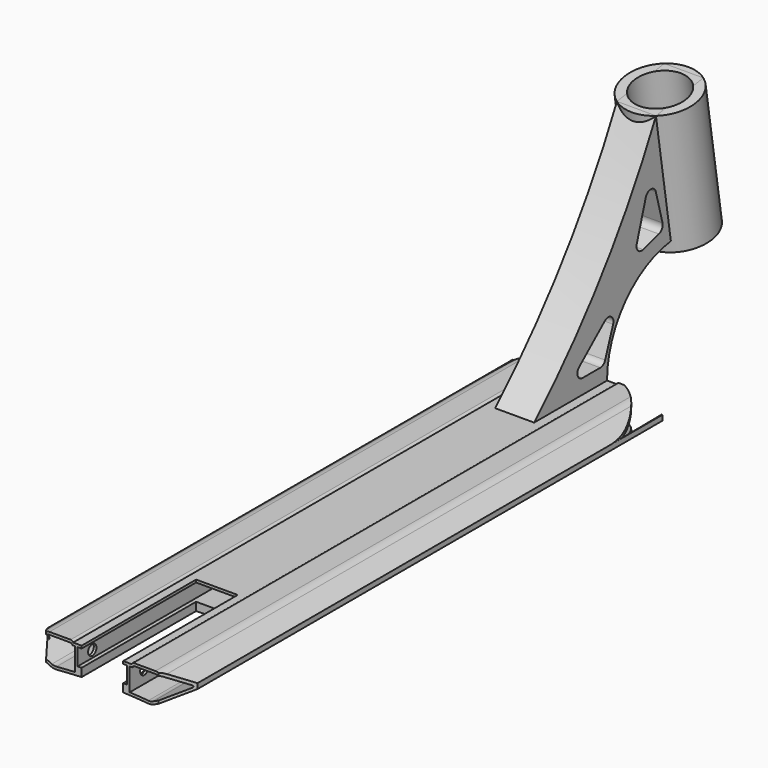
from build123d import *

# Parameters (mm, degrees)
F1_DEPTH       = 250
F2_W           = 38
F2_H           = 13
F3_DEPTH       = 250
F4_T1_DEPTH    = 509.3674969976
F5_R           = 9
F7_DEPTH       = 500.001
F9_DEPTH       = 0.9604886552
F9_DEPTH_BACK  = 22.8653446865
F11_DEPTH      = 0.9604887634
F11_DEPTH_BACK = 22.8653447865
F13_DEPTH      = 15
F14_R          = 27.5
F15_DEPTH      = 100
F17_D          = 40
F19_D          = 8
F19_DEPTH      = 78.501
F21_DEPTH      = 72.501


# Not quite as in the source:
# - a fillet or chamfer that OpenCascade refuses, or shapes differently, is made with other operations: its cross-section is extruded or revolved along the edge and cut away or added


with BuildPart() as f1:
    # F0 (on Front) → F1 (new body, symmetric)
    with BuildSketch(Plane.XZ):
        with BuildLine():
            Line((22.5, 21.5643446865), (0, 21.5643446865))
            Line((0, 21.5643446865), (-22.5, 21.5643446865))
            Line((-22.5, 21.5643446865), (-22.5, 22.8643446865))
            Line((-22.5, 22.8643446865), (-43.8217498065, 22.8643446865))
            Line((-43.8217498065, 22.8643446865), (-57.5, 12.151993139))
            Line((-57.5, 12.151993139), (-57.5, 8.151993139))
            Line((-57.5, 8.151993139), (-37.5, -1.1356553135))
            ThreePointArc((-37.5, -1.1356553135), (0, 0.564188832), (37.5, -1.1356553135))
            Line((37.5, -1.1356553135), (57.5, 8.151993139))
            Line((57.5, 8.151993139), (57.5, 12.151993139))
            Line((57.5, 12.151993139), (43.8217498065, 22.8643446865))
            Line((43.8217498065, 22.8643446865), (22.5, 22.8643446865))
            Line((22.5, 22.8643446865), (22.5, 21.5643446865))
        make_face()
    extrude(amount=F1_DEPTH, both=True)

    # F2 (on Front) → F3 (cut, symmetric)
    with BuildSketch(Plane.XZ):
        with Locations((0, 13.0643446865)):
            Rectangle(F2_W, F2_H)
    extrude(amount=F3_DEPTH, both=True, mode=Mode.SUBTRACT)

    # F4: fillet of radius 2 on 2 edges, made by hand

    # F4_s2 → F4_t1 (cut)
    with BuildSketch(Plane.XZ.offset(-254.6837484988)):
        with BuildLine():
            ThreePointArc((-24.3734993995, 22.8643446865), (-23.2333239744, 22.507512359), (-22.5, 21.5643446865))
            Line((-22.5, 21.5643446865), (-22.5, 22.8643446865))
            Line((-22.5, 22.8643446865), (-24.3734993995, 22.8643446865))
        make_face()
        with BuildLine():
            ThreePointArc((24.3734993995, 22.8643446865), (23.2333239744, 22.507512359), (22.5, 21.5643446865))
            Line((22.5, 21.5643446865), (22.5, 22.8643446865))
            Line((22.5, 22.8643446865), (24.3734993995, 22.8643446865))
        make_face()
    extrude(amount=F4_T1_DEPTH, mode=Mode.SUBTRACT)

    # F5
    f5_edges = [f1.edges().sort_by_distance(p)[0] for p in [
        (43.82175, 0, 22.864345),
        (-43.82175, 0, 22.864345),
        (-37.5, 0, -1.135655),
        (37.5, 0, -1.135655),
    ]]
    fillet(f5_edges, radius=F5_R)

    # F6 (on face) → F7 (cut, through all)
    with BuildSketch(Plane.XZ.offset(250)):
        with BuildLine():
            ThreePointArc((-38.8398592766, 1.6916831032), (-37.1099744385, 1.1473623621), (-35.2983129545, 1.0656966447))
            ThreePointArc((-35.2983129545, 1.0656966447), (-28.1533234397, 1.6115661831), (-21, 2.034428437))
            Line((-21, 2.034428437), (-21, 19.5643446865))
            Line((-21, 19.5643446865), (-23, 19.5643446865))
            ThreePointArc((-23, 19.5643446865), (-23.7333239744, 20.507512359), (-24.8734993995, 20.8643446865))
            Line((-24.8734993995, 20.8643446865), (-40.7169256034, 20.8643446865))
            ThreePointArc((-40.7169256034, 20.8643446865), (-42.9997645145, 20.4816437205), (-45.0329906666, 19.3753865454))
            Line((-45.0329906666, 19.3753865454), (-55.617097211, 11.0862656041))
            ThreePointArc((-55.617097211, 11.0862656041), (-55.9939317717, 10.1844048326), (-55.4216999505, 9.3919984469))
            Line((-55.4216999505, 9.3919984469), (-38.8398592766, 1.6916831032))
        make_face()
        with BuildLine():
            Line((21, 19.5643446865), (21, 2.034428437))
            ThreePointArc((21, 2.034428437), (28.1533234397, 1.6115661831), (35.2983129545, 1.0656966447))
            ThreePointArc((35.2983129545, 1.0656966447), (37.1099744385, 1.1473623621), (38.8398592766, 1.6916831032))
            Line((38.8398592766, 1.6916831032), (55.4216999505, 9.3919984469))
            ThreePointArc((55.4216999505, 9.3919984469), (55.9939317717, 10.1844048326), (55.617097211, 11.0862656041))
            Line((55.617097211, 11.0862656041), (45.0329906666, 19.3753865454))
            ThreePointArc((45.0329906666, 19.3753865454), (42.9997645145, 20.4816437205), (40.7169256034, 20.8643446865))
            Line((40.7169256034, 20.8643446865), (24.8734993995, 20.8643446865))
            ThreePointArc((24.8734993995, 20.8643446865), (23.7333239744, 20.507512359), (23, 19.5643446865))
            Line((23, 19.5643446865), (21, 19.5643446865))
        make_face()
    extrude(amount=-F7_DEPTH, mode=Mode.SUBTRACT)

    # F8 (on Top) → F9 (cut, two sides)
    with BuildSketch(Plane.XY) as f9_sk:
        with BuildLine():
            ThreePointArc((-57.4987473195, 200.3795480055), (0, 257.5), (57.4987473195, 200.3795480055))
            Line((57.4987473195, 200.3795480055), (56.9706690247, 280.3795480055))
            Line((56.9706690247, 280.3795480055), (-56.9706690247, 280.3795480055))
            Line((-56.9706690247, 280.3795480055), (-57.4987473195, 200.3795480055))
        make_face()
    extrude(amount=-F9_DEPTH, mode=Mode.SUBTRACT)
    extrude(f9_sk.sketch, amount=F9_DEPTH_BACK, mode=Mode.SUBTRACT)

    # F10 (on Top) → F11 (cut, two sides)
    with BuildSketch(Plane.XY) as f11_sk:
        Polygon((-16, -216.0670316956), (-43.2975540478, -216.0670316956), (-68, -182.0670316956), (-68, -312.0670316956), (0, -312.0670316956), (0, -106.0670316956), (-16, -106.0670316956), align=None)
        Polygon((16, -106.0670316956), (0, -106.0670316956), (0, -312.0670316956), (68, -312.0670316956), (68, -182.0670316956), (43.2975540478, -216.0670316956), (16, -216.0670316956), align=None)
    extrude(amount=-F11_DEPTH, mode=Mode.SUBTRACT)
    extrude(f11_sk.sketch, amount=F11_DEPTH_BACK, mode=Mode.SUBTRACT)

    # F12 (on Right) → F13 (join, symmetric)
    with BuildSketch(Plane.YZ):
        with BuildLine():
            ThreePointArc((297.0295354887, 181.5643446865), (245.7826981398, 96.2483289481), (180, 21.5643446865))
            Line((180, 21.5643446865), (250, 21.5643446865))
            ThreePointArc((250, 21.5643446865), (267.5395947829, 67.9098502341), (311.3687395561, 91.0301732869))
            Line((311.3687395561, 91.0301732869), (312.6729819927, 82.795510627))
            Line((312.6729819927, 82.795510627), (358.1066456601, 89.9914960188))
            Line((358.1066456601, 89.9914960188), (342.4631991561, 188.7603300783))
            Line((342.4631991561, 188.7603300783), (297.0295354887, 181.5643446865))
        make_face()
    extrude(amount=F13_DEPTH, both=True)

    # F14 (on face) → F15 (join, through all)
    with BuildSketch(Plane(origin=(0, -20.7844039253, 131.2275617651), x_dir=(1, 0, 0), z_dir=(0, -0.156434465, 0.9876883406))):
        with Locations((0, 344.775530146)):
            Circle(F14_R)
    extrude(amount=-F15_DEPTH)

    # F17 (through all)
    with Locations(Plane(origin=(0, -20.7844039253, 131.2275617651), x_dir=(1, 0, 0), z_dir=(0, -0.156434465, 0.9876883406))):
        with Locations((0, 344.775530146)):
            Hole(F17_D / 2)

    # F19 (through all, one way)
    with BuildSketch(Plane.YZ.offset(21)):
        with Locations((-202.0670316956, 12.034428437)):
            Circle(F19_D / 2)
    extrude(amount=-F19_DEPTH, mode=Mode.SUBTRACT)

    # F20 (on face) → F21 (cut, through all)
    with BuildSketch(Plane.YZ.offset(15)):
        with BuildLine():
            Line((303.3300998051, 106.5364009657), (296.8697635571, 130.2439192545))
            ThreePointArc((296.8697635571, 130.2439192545), (292.1354764945, 133.9285390129), (287.271901756, 130.4163406247))
            Line((287.271901756, 130.4163406247), (278.5350250255, 102.3679551307))
            ThreePointArc((278.5350250255, 102.3679551307), (279.7315404872, 97.3876414374), (284.6820479704, 96.0732406641))
            Line((284.6820479704, 96.0732406641), (299.8792609489, 100.4141078692))
            ThreePointArc((299.8792609489, 100.4141078692), (302.8617375272, 102.7667124398), (303.3300998051, 106.5364009657))
        make_face()
        with BuildLine():
            ThreePointArc((243.4909897109, 32.8643446865), (246.3588718926, 33.768584465), (248.1894528148, 36.1542439699))
            Line((248.1894528148, 36.1542439699), (255.8716915251, 57.2610213573))
            ThreePointArc((255.8716915251, 57.2610213573), (254.0207530146, 63.0810616952), (247.921439605, 62.7692623419))
            Line((247.921439605, 62.7692623419), (223.2683930345, 41.6624849544))
            ThreePointArc((223.2683930345, 41.6624849544), (221.8302617373, 36.1309522525), (226.5201818507, 32.8643446865))
            Line((226.5201818507, 32.8643446865), (243.4909897109, 32.8643446865))
        make_face()
    extrude(amount=-F21_DEPTH, mode=Mode.SUBTRACT)


solid = f1.part
